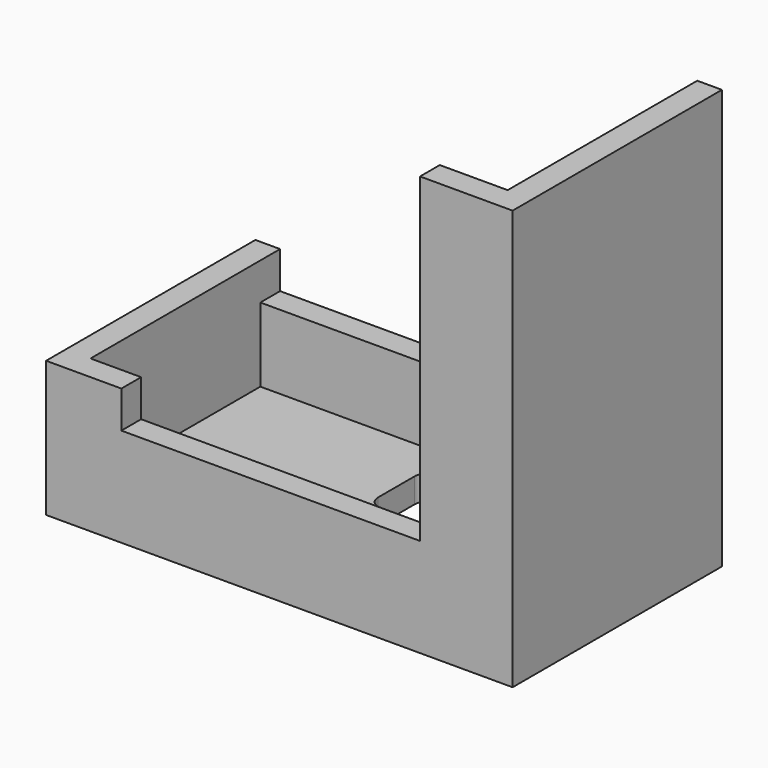
from build123d import *

# Parameters (mm, degrees)
F0_W      = 96.012
F0_H      = 86.36
F1_DEPTH  = 53.848
F2_T      = -5.08
F4_D      = 6.35
F6_DEPTH  = 25.4
F7_W      = 84.328
F7_H      = 66.04
F8_DEPTH  = 25.4
F9_W      = 53.848
F9_H      = 58.42
F10_DEPTH = 25.4
F11_W     = 85.852
F11_H     = 5.08
F12_DEPTH = 15.24
F13_DEPTH = 10.16
F14_DEPTH = 12.7


# Not quite as in the source:
# - a feature names something its author has since deleted; it is built from what else it names


with BuildPart() as f1:
    # F0 (on Front) → F1 (new body)
    with BuildSketch(Plane.XZ):
        with Locations((48.006, 43.18)):
            Rectangle(F0_W, F0_H)
    extrude(amount=F1_DEPTH)

    # F2
    f2_openings = [f1.faces().sort_by_distance(p)[0] for p in [
        (48.006, -26.924, 86.36),
        (48.006, 0, 43.18),
    ]]
    offset(amount=F2_T, openings=f2_openings)

    # F4 (through all)
    with Locations(Plane(origin=(0, 0, 0), x_dir=(1, 0, 0), z_dir=(0, 0, -1))):
        with Locations((17.018, 30.7086)):
            Hole(F4_D / 2)

    # F5 (on face) → F6 (cut)
    with BuildSketch(Plane(origin=(0, 0, 0), x_dir=(1, 0, 0), z_dir=(0, 0, -1))):
        with BuildLine():
            Line((76.962, 25.908), (46.482, 25.908))
            ThreePointArc((46.482, 25.908), (44.6859487758, 25.1640512242), (43.942, 23.368))
            Line((43.942, 23.368), (43.942, 13.97))
            ThreePointArc((43.942, 13.97), (44.6859487758, 12.1739487758), (46.482, 11.43))
            Line((46.482, 11.43), (76.962, 11.43))
            ThreePointArc((76.962, 11.43), (78.7580512242, 12.1739487758), (79.502, 13.97))
            Line((79.502, 13.97), (79.502, 23.368))
            ThreePointArc((79.502, 23.368), (78.7580512242, 25.1640512242), (76.962, 25.908))
        make_face()
    extrude(amount=-F6_DEPTH, mode=Mode.SUBTRACT)

    # F7 (on face) → F8 (cut)
    with BuildSketch(Plane.XZ.offset(53.848)):
        with Locations((47.498, 53.34)):
            Rectangle(F7_W, F7_H)
    extrude(amount=-F8_DEPTH, mode=Mode.SUBTRACT)

    # F9 (on face) → F10 (cut)
    with BuildSketch(Plane(origin=(0, 0, 0), x_dir=(0, -1, 0), z_dir=(-1, 0, 0))):
        with Locations((26.924, 57.15)):
            Rectangle(F9_W, F9_H)
    extrude(amount=-F10_DEPTH, mode=Mode.SUBTRACT)

    # F11 (on face) → F12 (join)
    with BuildSketch(Plane.XY.offset(5.08)):
        with Locations((48.006, -2.54)):
            Rectangle(F11_W, F11_H)
    extrude(amount=F12_DEPTH)

    # F13 (add): a face of the model
    f13_faces = [f1.faces().sort_by_distance(p)[0] for p in [
        (5.334, -51.308, 24.13),
    ]]
    extrude(f13_faces, amount=F13_DEPTH)

    # F14 (add): a face of the model
    f14_faces = [f1.faces().sort_by_distance(p)[0] for p in [
        (89.662, -51.308, 53.34),
    ]]
    extrude(f14_faces, amount=F14_DEPTH)


solid = f1.part
